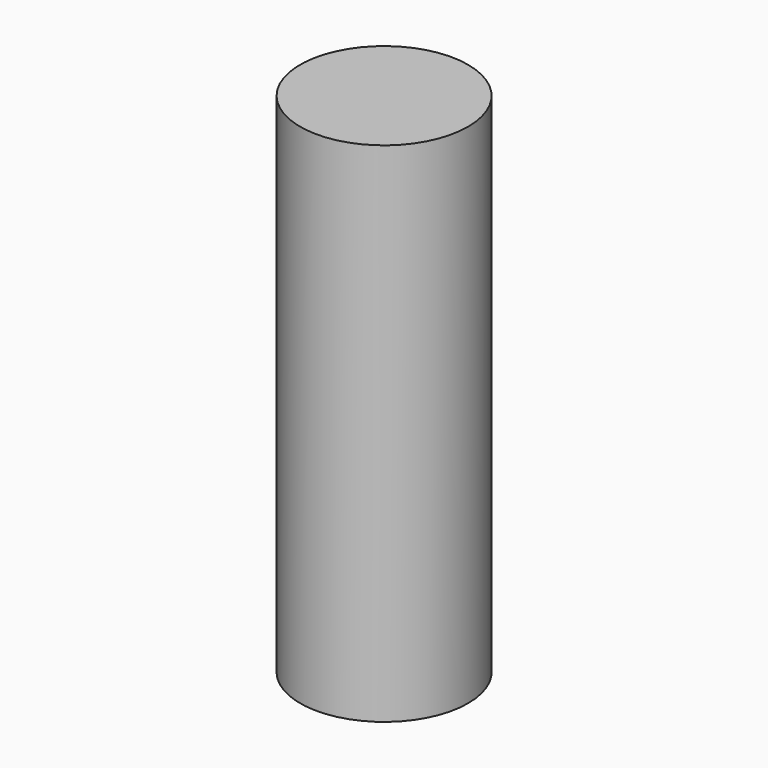
from build123d import *

# Parameters (mm, degrees)
F0_R     = 22.5
F1_DEPTH = 68
F2_R     = 3
F3_DEPTH = 1.1


# Not quite as in the source:
# - the program builds the solid bodies; features that only make, move or delete a surface that nothing else refers to are left out


with BuildPart() as f1:
    # F0 (on Top) → F1 (new body, symmetric)
    with BuildSketch(Plane.XY):
        Circle(F0_R)
    extrude(amount=F1_DEPTH, both=True)


with BuildPart() as f3:
    # F2 (on Front) → F3 (new body, symmetric)
    with BuildSketch(Plane.XZ):
        with Locations((-23.4349872917, 54.1538223624)):
            Circle(F2_R)
    extrude(amount=F3_DEPTH, both=True)


solid = Compound([f1.part, f3.part])
